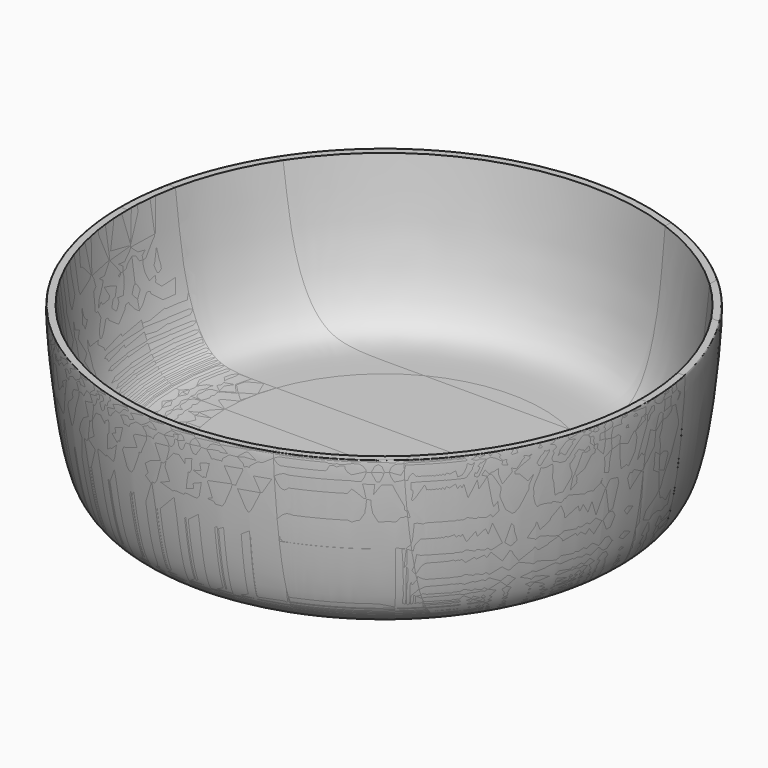
from build123d import *

# Parameters (mm, degrees)
F0_W      = 100
F0_H      = 35
F1_DEPTH  = 50
F0_W_2    = 25
F2_DEPTH  = 50
F0_W_3    = 35
F3_DEPTH  = 50
F4_DEPTH  = 50
F0_H_2    = 15
F0_H_3    = 75
F5_DEPTH  = 50
F6_DEPTH  = 50
F7_DEPTH  = 50
F8_DEPTH  = 50
F9_DEPTH  = 50
F10_DEPTH = 50
F11_DEPTH = 50
F12_DEPTH = 50
F13_W     = 25
F13_H     = 4.0908760428


# Not quite as in the source:
# - a feature names something its author has since deleted; it is built from what else it names


with BuildPart() as f1:
    # F0 (on Top) → F1 (new body)
    with BuildSketch(Plane.XY):
        with Locations((50, 42.5)):
            Rectangle(F0_W, F0_H)
    extrude(amount=F1_DEPTH)


with BuildPart() as f2:
    # F0 (on Top) → F2 (new body)
    with BuildSketch(Plane.XY):
        with Locations((112.5, 42.5)):
            Rectangle(F0_W_2, F0_H)
    extrude(amount=F2_DEPTH)


with BuildPart() as f3:
    # F0 (on Top) → F3 (new body)
    with BuildSketch(Plane.XY):
        with Locations((142.5, 42.5)):
            Rectangle(F0_W_3, F0_H)
    extrude(amount=F3_DEPTH)


with BuildPart() as f4:
    # F0 (on Top) → F4 (new body)
    with BuildSketch(Plane.XY):
        Polygon((0, 25), (0, 0), (100, 0), (125, 0), (160, 0), (160, 25), (125, 25), (100, 25), align=None)
    extrude(amount=F4_DEPTH)


with BuildPart() as f5:
    # F0 (on Top) → F5 (new body)
    with BuildSketch(Plane.XY):
        with Locations((50, -7.5)):
            Rectangle(F0_W, F0_H_2)
        with Locations((50, -52.5)):
            Rectangle(F0_W, F0_H_3)
    extrude(amount=F5_DEPTH)


with BuildPart() as f5b:
    # F0 (on Top) → F5, piece 2 (new body)
    with BuildSketch(Plane.XY):
        with Locations((142.5, -7.5)):
            Rectangle(F0_W_3, F0_H_2)
        with Locations((142.5, -52.5)):
            Rectangle(F0_W_3, F0_H_3)
    extrude(amount=F5_DEPTH)


with BuildPart() as f6:
    # F0 (on Top) → F6 (new body)
    with BuildSketch(Plane.XY):
        with Locations((112.5, -7.5)):
            Rectangle(F0_W_2, F0_H_2)
        with Locations((112.5, -52.5)):
            Rectangle(F0_W_2, F0_H_3)
    extrude(amount=F6_DEPTH)


with BuildPart() as f7:
    # F0 (on Top) → F7 (new body)
    with BuildSketch(Plane.XY):
        with Locations((50, -7.5)):
            Rectangle(F0_W, F0_H_2)
    extrude(amount=F7_DEPTH)


with BuildPart() as f8:
    # F0 (on Top) → F8 (new body)
    with BuildSketch(Plane.XY):
        with Locations((112.5, -7.5)):
            Rectangle(F0_W_2, F0_H_2)
    extrude(amount=F8_DEPTH)


with BuildPart() as f9:
    # F0 (on Top) → F9 (new body)
    with BuildSketch(Plane.XY):
        with Locations((142.5, -7.5)):
            Rectangle(F0_W_3, F0_H_2)
    extrude(amount=F9_DEPTH)


with BuildPart() as f10:
    # F0 (on Top) → F10 (new body)
    with BuildSketch(Plane.XY):
        with Locations((50, -52.5)):
            Rectangle(F0_W, F0_H_3)
    extrude(amount=F10_DEPTH)


with BuildPart() as f11:
    # F0 (on Top) → F11 (new body)
    with BuildSketch(Plane.XY):
        with Locations((112.5, -52.5)):
            Rectangle(F0_W_2, F0_H_3)
    extrude(amount=F11_DEPTH)


with BuildPart() as f12:
    # F0 (on Top) → F12 (new body)
    with BuildSketch(Plane.XY):
        with Locations((142.5, -52.5)):
            Rectangle(F0_W_3, F0_H_3)
    extrude(amount=F12_DEPTH)


with BuildPart() as f14_tool:
    # F13 (on face) → F14 (revolve)
    with BuildSketch(Plane.XZ.offset(15)):
        with Locations((87.5, 6.0454380214)):
            Rectangle(F13_W, F13_H)
        with BuildLine():
            Line((100, 8.0908760428), (100, 4))
            Line((100, 4), (101, 4))
            Line((101, 4), (100, 1.7719826878))
            Line((100, 1.7719826878), (100, 0))
            Line((100, 0), (119.2046818137, 0))
            add(Edge.make_bspline(
                [(119.2046818137, 0), (126.2493979814, 0.7732794744), (138.9863898746, 2.1713846872), (147.3157369656, 10.0187020689), (150.1161102275, 49.1551977245), (149.4910913046, 48.7744319361), (149.4630426168, 48.7573444843)],
                knots=[0, 0, 0, 0, 0.3078185803, 0.5565423317, 0.9800991534, 1, 1, 1, 1], degree=3))
            Line((149.4630426168, 48.7573444843), (147.5605070591, 48.7573444843))
            add(Edge.make_bspline(
                [(120, 8.0908760428), (129.3039530386, 8.0908760428), (138.5548123003, 7.3831138404), (145.7109533824, 27.1683688424), (146.7088145562, 41.5130421868), (147.5605070591, 48.7573444843)],
                knots=[0, 0, 0, 0, 0.3205308098, 0.6379484552, 1, 1, 1, 1], degree=3))
            Line((120, 8.0908760428), (100, 8.0908760428))
        make_face()
        Polygon((100, 0), (100, 1.7719826878), (99.2046818137, 0), align=None)
    revolve(axis=Axis((75, -15, 22.4669491872), (0, 0, -1)))


with BuildPart() as f1_1:
    add(f1.part)

    # F14: intersect by f14_tool
    add(f14_tool.part, mode=Mode.INTERSECT)


with BuildPart() as f2_1:
    add(f2.part)

    # F14: intersect by f14_tool
    add(f14_tool.part, mode=Mode.INTERSECT)


with BuildPart() as f3_1:
    add(f3.part)

    # F14: intersect by f14_tool
    add(f14_tool.part, mode=Mode.INTERSECT)


with BuildPart() as f4_1:
    add(f4.part)

    # F14: intersect by f14_tool
    add(f14_tool.part, mode=Mode.INTERSECT)


with BuildPart() as f5_1:
    add(f5.part)

    # F14: intersect by f14_tool
    add(f14_tool.part, mode=Mode.INTERSECT)


with BuildPart() as f5b_1:
    add(f5b.part)

    # F14: intersect by f14_tool
    add(f14_tool.part, mode=Mode.INTERSECT)


with BuildPart() as f6_1:
    add(f6.part)

    # F14: intersect by f14_tool
    add(f14_tool.part, mode=Mode.INTERSECT)


with BuildPart() as f7_1:
    add(f7.part)

    # F14: intersect by f14_tool
    add(f14_tool.part, mode=Mode.INTERSECT)


with BuildPart() as f8_1:
    add(f8.part)

    # F14: intersect by f14_tool
    add(f14_tool.part, mode=Mode.INTERSECT)


with BuildPart() as f9_1:
    add(f9.part)

    # F14: intersect by f14_tool
    add(f14_tool.part, mode=Mode.INTERSECT)


with BuildPart() as f10_1:
    add(f10.part)

    # F14: intersect by f14_tool
    add(f14_tool.part, mode=Mode.INTERSECT)


with BuildPart() as f11_1:
    add(f11.part)

    # F14: intersect by f14_tool
    add(f14_tool.part, mode=Mode.INTERSECT)


with BuildPart() as f12_1:
    add(f12.part)

    # F14: intersect by f14_tool
    add(f14_tool.part, mode=Mode.INTERSECT)


solid = Compound([f1_1.part, f2_1.part, f3_1.part, f4_1.part, f5_1.part, f5b_1.part, f6_1.part, f7_1.part, f8_1.part, f9_1.part, f10_1.part, f11_1.part, f12_1.part])
